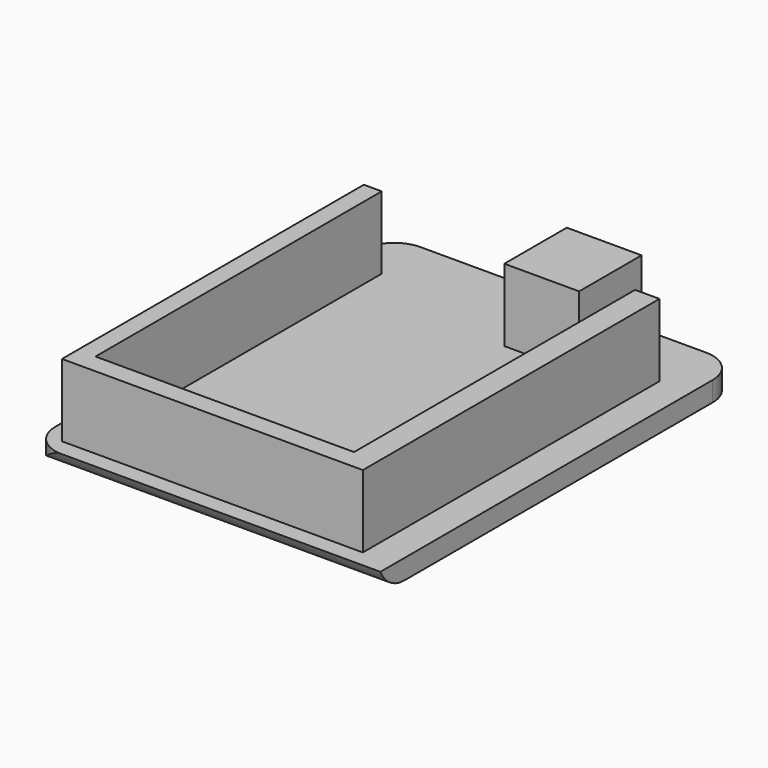
from build123d import *

# Parameters (mm, degrees)
F1_DEPTH    = 14
F0_W        = 11.3450561184
F0_H        = 11.8383169174
F0_W_2      = 53.3
F0_H_2      = 68
F2_DEPTH    = 3
F3_T1_DEPTH = 28
F3_T3_DEPTH = 76.2128784748


# Not quite as in the source:
# - a fillet or chamfer that OpenCascade refuses, or shapes differently, is made with other operations: its cross-section is extruded or revolved along the edge and cut away or added


with BuildPart() as f1:
    # F0 (on Top) → F1 (new body)
    with BuildSketch(Plane.XY):
        Polygon((-20.2707853168, 36.2087599933), (-22.9837335646, 36.2087599933), (-22.9837335646, -18.0502012372), (-22.9837335646, -21.0097823292), (-20.2707853168, -21.0097823292), (18.9436431974, -21.0097823292), (22.6431209594, -21.0097823292), (22.6431209594, -18.0502012372), (22.6431209594, 35.2222323418), (18.9436431974, 35.2222323418), (18.9436431974, -18.0502012372), (-20.2707853168, -18.0502012372), align=None)
    extrude(amount=F1_DEPTH)



with BuildPart() as f1b:
    # F0 (on Top) → F1, piece 2 (new body)
    with BuildSketch(Plane.XY):
        with Locations((8.338484331, 36.7020219564)):
            Rectangle(F0_W, F0_H)
    extrude(amount=F1_DEPTH)


with BuildPart() as f1_1:
    add(f1.part)

    add(f1b.part)  # F2 merges F1b
    # F0 (on Top) → F2 (join)
    with BuildSketch(Plane.XY):
        with Locations((0.7177972624, 10.4120122269)):
            Rectangle(F0_W_2, F0_H_2)
        Polygon((-22.9837335646, -18.0502012372), (-22.9837335646, 36.2087599933), (-20.2707853168, 36.2087599933), (-20.2707853168, -18.0502012372), (18.9436431974, -18.0502012372), (18.9436431974, 35.2222323418), (22.6431209594, 35.2222323418), (22.6431209594, -18.0502012372), (22.6431209594, -21.0097823292), (18.9436431974, -21.0097823292), (-20.2707853168, -21.0097823292), (-22.9837335646, -21.0097823292), align=None, mode=Mode.SUBTRACT)
        with Locations((8.338484331, 36.7020219564)):
            Rectangle(F0_W, F0_H, mode=Mode.SUBTRACT)
    extrude(amount=F2_DEPTH)

    # F3: fillet of radius 5 on 4 edges, made by hand

    # F3_s2 → F3_t1 (cut)
    with BuildSketch(Plane.XY.offset(-12.5)):
        with BuildLine():
            ThreePointArc((-20.9322027376, 44.4120122269), (-24.4677366436, 42.9475461328), (-25.9322027376, 39.4120122269))
            Line((-25.9322027376, 39.4120122269), (-25.9322027376, 44.4120122269))
            Line((-25.9322027376, 44.4120122269), (-20.9322027376, 44.4120122269))
        make_face()
        with BuildLine():
            ThreePointArc((-25.9322027376, -18.5879877731), (-24.4677366436, -22.1235216791), (-20.9322027376, -23.5879877731))
            Line((-20.9322027376, -23.5879877731), (-25.9322027376, -23.5879877731))
            Line((-25.9322027376, -23.5879877731), (-25.9322027376, -18.5879877731))
        make_face()
        with BuildLine():
            ThreePointArc((22.3677972624, 44.4120122269), (25.9033311683, 42.9475461328), (27.3677972624, 39.4120122269))
            Line((27.3677972624, 39.4120122269), (27.3677972624, 44.4120122269))
            Line((27.3677972624, 44.4120122269), (22.3677972624, 44.4120122269))
        make_face()
    extrude(amount=F3_T1_DEPTH, mode=Mode.SUBTRACT)

    # F3_s4 → F3_t3 (cut)
    with BuildSketch(Plane.YZ.offset(-37.388641975)):
        with BuildLine():
            ThreePointArc((-23.5879877731, 3), (-21.7440248657, 0.8166998673), (-19.0054120782, 0))
            Line((-19.0054120782, 0), (-23.5879877731, 0))
            Line((-23.5879877731, 0), (-23.5879877731, 3))
        make_face()
    extrude(amount=F3_T3_DEPTH, mode=Mode.SUBTRACT)


solid = f1_1.part
